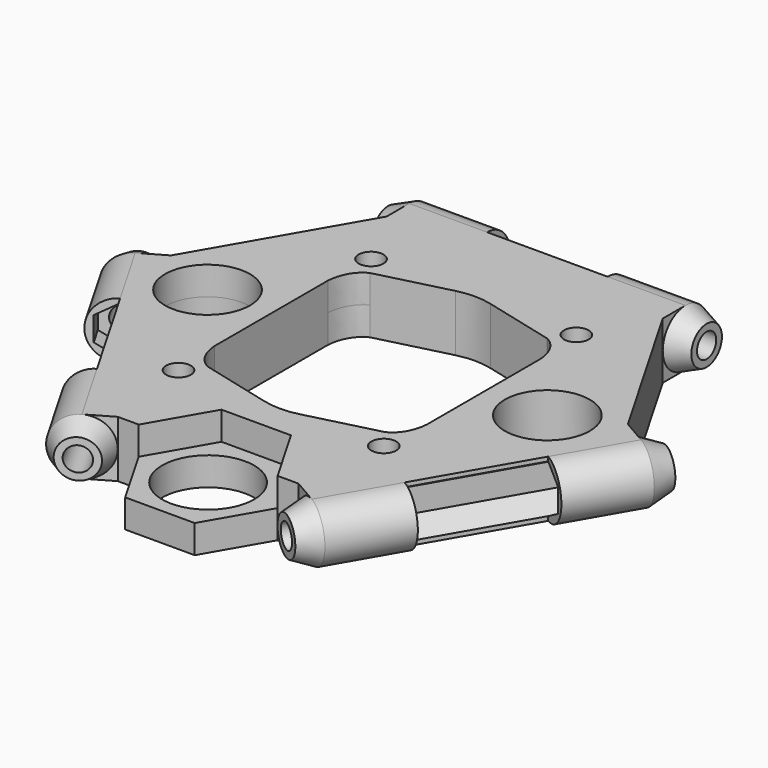
from build123d import *

# Parameters (mm, degrees)
F4_DEPTH  = 19.5
F5_DEPTH  = 4
F6_DEPTH  = 11.5
F7_DEPTH  = 8.5
F9_COUNT  = 3
F9_ANGLE  = 240
F2_R      = 1.75
F2_R_2    = 6
F10_DEPTH = 4
F11_R     = 6.5
F12_DEPTH = 20
F13_DEPTH = 4


# Not quite as in the source:
# - a feature of the source that left no trace in its solid (it failed there, or was rolled back) is left out
# - a feature names something its author has since deleted; it is built from what else it names


with BuildPart() as f3:
    # F0 (on Top) → F3 (revolve)
    with BuildSketch(Plane.XY):
        Polygon((19.5, 34), (0, 34), (0, 31.7), (22.5, 31.7), (22.5, 32.7), align=None)
    revolve(axis=Axis((11.25, 30, 0), (1, 0, 0)))

    # F1 (on Right) → F4 (join)
    with BuildSketch(Plane.YZ):
        with BuildLine():
            Line((26, 4), (26, 0))
            ThreePointArc((26, 0), (27.1715728753, 2.8284271247), (30, 4))
            Line((30, 4), (26, 4))
        make_face()
        with BuildLine():
            Line((26, -4), (30, -4))
            ThreePointArc((30, -4), (27.1715728753, -2.8284271247), (26, 0))
            Line((26, 0), (26, -4))
        make_face()
    extrude(amount=F4_DEPTH)

    # F0 (on Top) → F5 (join, symmetric)
    with BuildSketch(Plane.XY):
        Polygon((19.5, 26), (0, 26), (0, 0), (25.8833302492, 14.9437476869), align=None)
    extrude(amount=F5_DEPTH, both=True)

    # F1 (on Right) → F6 (cut)
    with BuildSketch(Plane.YZ):
        Polygon((30, -3.4063665882), (32.95, -1.7031832941), (32.95, 1.7031832941), (30, 3.4063665882), (27.05, 1.7031832941), (27.05, -1.7031832941), align=None)
    extrude(amount=F6_DEPTH, mode=Mode.SUBTRACT)

    # F1 (on Right) → F7 (cut)
    with BuildSketch(Plane.YZ):
        with BuildLine():
            Line((32.95, 1.7031832941), (32.95, -1.7031832941))
            Line((32.95, -1.7031832941), (30, -3.4063665882))
            Line((30, -3.4063665882), (30, -4))
            ThreePointArc((30, -4), (32.8284271247, -2.8284271247), (34, 0))
            ThreePointArc((34, 0), (32.8284271247, 2.8284271247), (30, 4))
            Line((30, 4), (30, 3.4063665882))
            Line((30, 3.4063665882), (32.95, 1.7031832941))
        make_face()
    extrude(amount=F7_DEPTH, mode=Mode.SUBTRACT)

    # F8: F3 across plane


with BuildPart() as f3_1:
    add(f3.part)
    add(f3.part.mirror(Plane.YZ))

    # F9: F3 ×3 about axis
    f9_axis = Axis((0, 0, 0), (0, 0, -1))


with BuildPart() as f3_2:
    add(f3_1.part)
    for i in range(1, F9_COUNT):
        add(f3_1.part.rotate(f9_axis, i * F9_ANGLE / (F9_COUNT - 1)))

    # F2 (on Top) → F10 (cut, symmetric)
    with BuildSketch(Plane.XY):
        with Locations((14.5, 17)):
            Circle(F2_R)
        with BuildLine():
            add(Edge.make_bspline(
                [(12.5257586532, 14.3151527465), (13.3123168346, 13.9246002449), (14.4418337404, 12.6938657), (14.9288469383, 11.0046443666), (15, 10)],
                knots=[0, 0, 0, 0, 0.4852212686, 1, 1, 1, 1], degree=3))
            Line((12.5257586532, 14.3151527465), (2.4642293228, 16.8734356371))
            ThreePointArc((2.4642293228, 16.8734356371), (0, 17.1818117358), (-2.4642293228, 16.8734356371))
            Line((-2.4642293228, 16.8734356371), (-12.5257586532, 14.3151527465))
            add(Edge.make_bspline(
                [(-12.5257586532, 14.3151527465), (-13.3123168346, 13.9246002449), (-14.4418337404, 12.6938657), (-14.9288469383, 11.0046443666), (-15, 10)],
                knots=[0, 0, 0, 0, 0.4852212686, 1, 1, 1, 1], degree=3))
            Line((-15, 10), (-15, 0))
            Line((-15, 0), (-15, -10))
            add(Edge.make_bspline(
                [(-12.5257586532, -14.3151527465), (-13.3123168346, -13.9246002449), (-14.4418337404, -12.6938657), (-14.9288469383, -11.0046443666), (-15, -10)],
                knots=[0, 0, 0, 0, 0.4852212686, 1, 1, 1, 1], degree=3))
            Line((-12.5257586532, -14.3151527465), (-2.4642293228, -16.8734356371))
            ThreePointArc((-2.4642293228, -16.8734356371), (0, -17.1818117358), (2.4642293228, -16.8734356371))
            Line((2.4642293228, -16.8734356371), (12.5257586532, -14.3151527465))
            add(Edge.make_bspline(
                [(12.5257586532, -14.3151527465), (13.3123168346, -13.9246002449), (14.4418337404, -12.6938657), (14.9288469383, -11.0046443666), (15, -10)],
                knots=[0, 0, 0, 0, 0.4852212686, 1, 1, 1, 1], degree=3))
            Line((15, -10), (15, 0))
            Line((15, 0), (15, 10))
        make_face()
        with Locations((-14.5, 17)):
            Circle(F2_R)
        with Locations((-14.5, -17)):
            Circle(F2_R)
        with Locations((14.5, -17)):
            Circle(F2_R)
        with Locations((-24, 0)):
            Circle(F2_R_2)
        with Locations((24, 0)):
            Circle(F2_R_2)
    extrude(amount=F10_DEPTH, both=True, mode=Mode.SUBTRACT)

    # F11 (on Top) → F12 (cut, symmetric)
    with BuildSketch(Plane.XY):
        Polygon((4.9074772881, -21.4), (-4.9074772881, -21.4), (-9.8149545762, -29.9), (-4.9074772881, -38.4), (4.9074772881, -38.4), (9.8149545762, -29.9), align=None)
        with Locations((0, -29.9)):
            Circle(F11_R, mode=Mode.SUBTRACT)
        with Locations((0, -29.9)):
            Circle(F11_R)
    extrude(amount=F12_DEPTH, both=True, mode=Mode.SUBTRACT)

    # F11 (on Top) → F13 (join)
    with BuildSketch(Plane.XY):
        Polygon((4.9074772881, -21.4), (-4.9074772881, -21.4), (-9.8149545762, -29.9), (-4.9074772881, -38.4), (4.9074772881, -38.4), (9.8149545762, -29.9), align=None)
        with Locations((0, -29.9)):
            Circle(F11_R, mode=Mode.SUBTRACT)
    extrude(amount=-F13_DEPTH)


solid = f3_2.part
